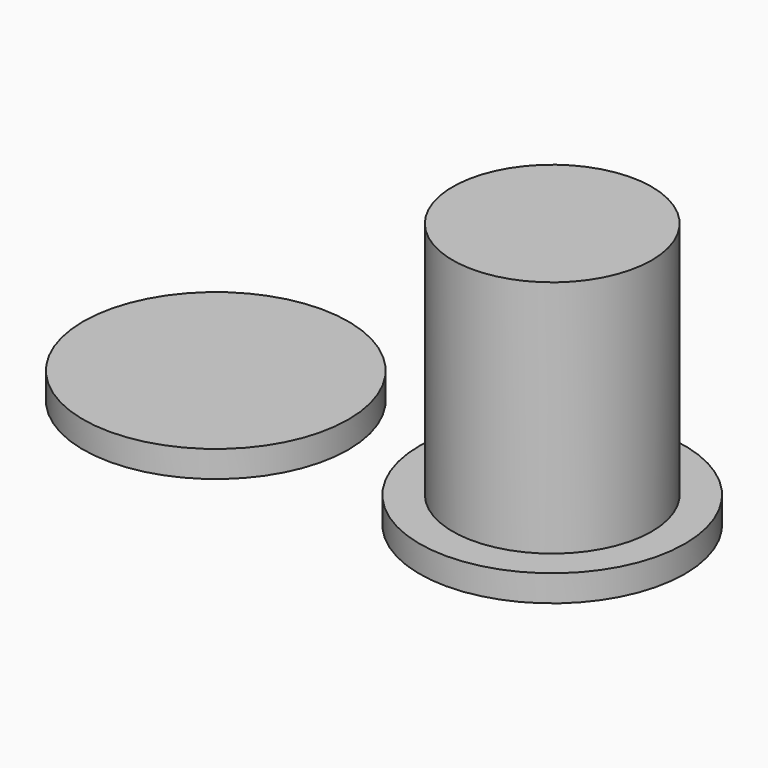
from build123d import *

# Parameters (mm, degrees)
F0_R     = 10
F1_DEPTH = 2
F2_R     = 7.5
F3_DEPTH = 20


# Not quite as in the source:
# - the program builds the solid bodies; features that only make, move or delete a surface that nothing else refers to are left out


with BuildPart() as f1:
    # F0 (on Top) → F1 (new body)
    with BuildSketch(Plane.XY):
        Circle(F0_R)
    extrude(amount=F1_DEPTH)

    # F2 (on Top) → F3 (join)
    with BuildSketch(Plane.XY):
        Circle(F2_R)
    extrude(amount=F3_DEPTH)


with BuildPart() as f1b:
    # F0 (on Top) → F1, piece 2 (new body)
    with BuildSketch(Plane.XY):
        with Locations((-25.3602210878, 0)):
            Circle(F0_R)
    extrude(amount=F1_DEPTH)


solid = Compound([f1.part, f1b.part])
